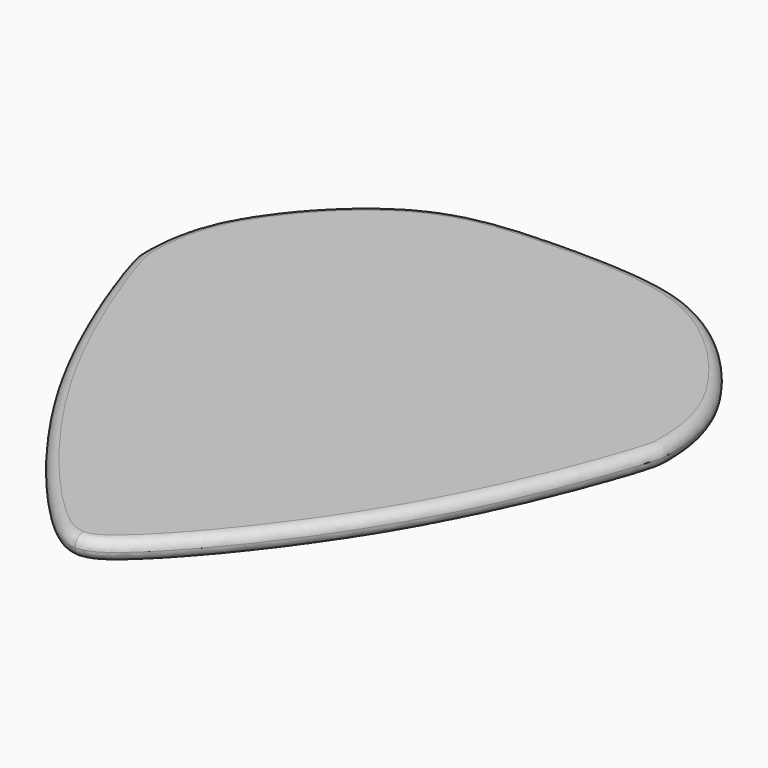
from build123d import *

# Parameters (mm, degrees)
F1_DEPTH = 1
F2_R     = 0.49999


# Not quite as in the source:
# - a fillet or chamfer is up to 0.001 mm smaller than in the source, because OpenCascade refuses the exact size


with BuildPart() as f1:
    # F0 (on Top) → F1 (new body)
    with BuildSketch(Plane.XY):
        with BuildLine():
            Line((-26, 21), (-13, 21))
            Line((-13, 21), (-13, 31.5220170279))
            add(Edge.make_bspline(
                [(-26, 21), (-26, 23.0869125682), (-24.8783342178, 26.2396543469), (-19.6697275677, 31.4126062683), (-15.3582775965, 31.5024927258), (-13, 31.5220170279)],
                knots=[0, 0, 0, 0, 0.3108261295, 0.6565499036, 1, 1, 1, 1], degree=3))
        make_face()
        with BuildLine():
            Line((-13, 21), (0, 21))
            add(Edge.make_bspline(
                [(0, 21), (0, 23.0869125682), (-1.1216657822, 26.2396543469), (-6.3302724323, 31.4126062683), (-10.6417224035, 31.5024927258), (-13, 31.5220170279)],
                knots=[0, 0, 0, 0, 0.3108261295, 0.6565499036, 1, 1, 1, 1], degree=3))
            Line((-13, 31.5220170279), (-13, 21))
        make_face()
        with BuildLine():
            add(Edge.make_bspline(
                [(-26, 21), (-26, 20.7234602422), (-25.9861320118, 20.1880475794), (-22.4175713066, 9.7994858104), (-14.5955903728, 0.788845571), (-13.3093070088, 0.621737619), (-13, 0.5861966638)],
                knots=[0, 0, 0, 0, 0.097446506, 0.4748377135, 0.875125803, 1, 1, 1, 1], degree=3))
            Line((-13, 0.5861966638), (-13, 21))
            Line((-13, 21), (-26, 21))
        make_face()
        with BuildLine():
            add(Edge.make_bspline(
                [(0, 21), (0, 20.7234602422), (-0.0138679882, 20.1880475794), (-3.5824286934, 9.7994858104), (-11.4044096272, 0.788845571), (-12.6906929912, 0.621737619), (-13, 0.5861966638)],
                knots=[0, 0, 0, 0, 0.097446506, 0.4748377135, 0.875125803, 1, 1, 1, 1], degree=3))
            Line((0, 21), (-13, 21))
            Line((-13, 21), (-13, 0.5861966638))
        make_face()
    extrude(amount=F1_DEPTH)

    # F2 (radius 0.5 in the source; OpenCascade refuses exactly that, so slightly less here)
    f2_edges = [f1.edges().sort_by_distance(p)[0] for p in [
        (-25.198327, 18.09063, 1),
        (-0.801673, 18.09063, 1),
        (-25.198327, 18.09063, 0),
        (-0.801673, 18.09063, 0),
    ]]
    fillet(f2_edges, radius=F2_R)


solid = f1.part
